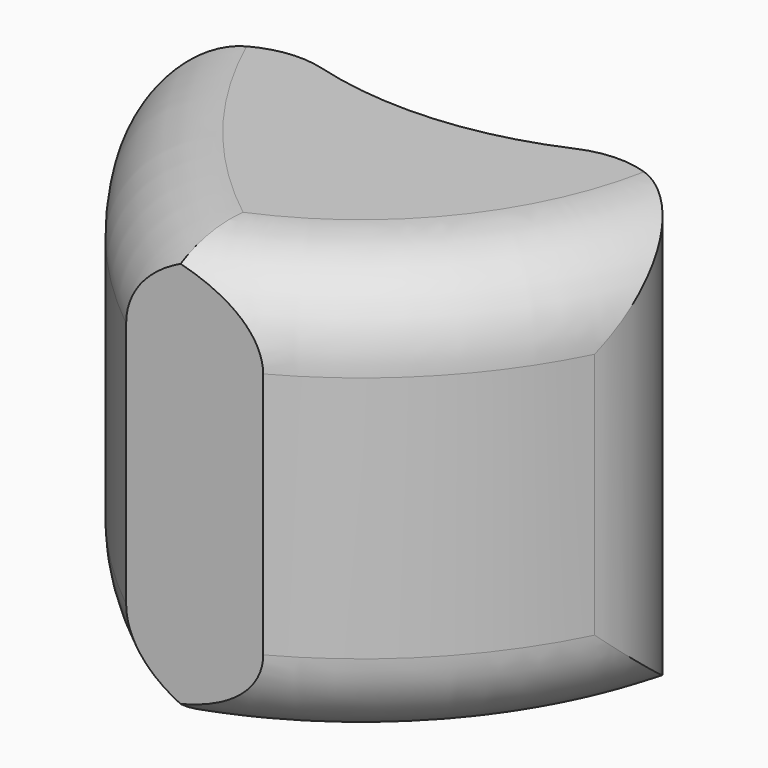
from build123d import *

# Parameters (mm, degrees)
F1_DEPTH     = 23.876
F2_T1_DEPTH  = 110.599658452
F2_T3_DEPTH  = 97.7290207292
F2_T6_ANGLE  = 84.0775345573
F2_T8_ANGLE  = 131.5876567491
F2_T10_ANGLE = 131.5876567491
F2_T12_ANGLE = 84.0775345573


# Not quite as in the source:
# - a fillet or chamfer that OpenCascade refuses, or shapes differently, is made with other operations: its cross-section is extruded or revolved along the edge and cut away or added


with BuildPart() as f1:
    # F0 (on Top) → F1 (new body)
    with BuildSketch(Plane.XY):
        with BuildLine():
            ThreePointArc((-16.8886538595, 0), (-33.6717544124, -9.3917342028), (-50.4548549652, 0))
            ThreePointArc((-50.4548549652, 0), (-46.0831484668, -13.8741388275), (-36.7328226566, -25.0175204128))
            Line((-36.7328226566, -25.0175204128), (-29.1329286993, -25.0175204128))
            ThreePointArc((-29.1329286993, -25.0175204128), (-19.0105144226, -14.4666076853), (-16.8886538595, 0))
        make_face()
    extrude(amount=-F1_DEPTH)

    # F2: fillet of radius 5.08 on 6 edges, made by hand

    # F2_s2 → F2_t1 (cut)
    with BuildSketch(Plane.XY.offset(-67.237829226)):
        with BuildLine():
            ThreePointArc((-38.9861518203, -8.6610502297), (-44.4536744732, -10.5484087098), (-44.6103785769, -16.3303953767))
            ThreePointArc((-44.6103785769, -16.3303953767), (-48.4959513119, -8.5099649673), (-50.4548549652, 0))
            ThreePointArc((-50.4548549652, 0), (-45.5388644987, -5.4141743653), (-38.9861518203, -8.6610502297))
        make_face()
    extrude(amount=F2_T1_DEPTH, mode=Mode.SUBTRACT)

    # F2_s4 → F2_t3 (cut)
    with BuildSketch(Plane.XY.offset(-60.8025103646)):
        with BuildLine():
            ThreePointArc((-19.0798772238, -14.6071656046), (-19.9573949525, -8.8324154802), (-25.6877196822, -7.7005343667))
            ThreePointArc((-25.6877196822, -7.7005343667), (-20.7034351336, -4.5184374558), (-16.8886538595, 0))
            ThreePointArc((-16.8886538595, 0), (-16.8326353552, -7.4763390399), (-19.0798772238, -14.6071656046))
        make_face()
    extrude(amount=F2_T3_DEPTH, mode=Mode.SUBTRACT)

    # F2_s5 → F2_t6 (revolve, cut)
    with BuildSketch(Plane(origin=(0.1965344141, 0.8317793395, 0), x_dir=(0, 0, 1), z_dir=(0.2299501287, 0.9732024138, 0))):
        with BuildLine():
            ThreePointArc((-5.08, -51.2464457493), (-1.4878975516, -49.7585481977), (0, -46.1664457493))
            Line((0, -46.1664457493), (0, -51.2464457493))
            Line((0, -51.2464457493), (-5.08, -51.2464457493))
        make_face()
    revolve(axis=Axis((-13.4102859167, 4.0468248863, 0), (0, 0, 1)), revolution_arc=F2_T6_ANGLE, mode=Mode.SUBTRACT)

    # F2_s7 → F2_t8 (revolve, cut)
    with BuildSketch(Plane(origin=(-40.3967670298, 1.3205110393, 0), x_dir=(0, 0, 1), z_dir=(-0.9994661577, 0.0326710822, 0))):
        with BuildLine():
            ThreePointArc((-5.08, -29.2399824093), (-1.4878975516, -27.7520848577), (0, -24.1599824093))
            Line((0, -24.1599824093), (0, -29.2399824093))
            Line((0, -29.2399824093), (-5.08, -29.2399824093))
        make_face()
    revolve(axis=Axis((-40.5679344471, -3.9158028389, 0), (0, 0, 1)), revolution_arc=F2_T8_ANGLE, mode=Mode.SUBTRACT)

    # F2_s9 → F2_t10 (revolve, cut)
    with BuildSketch(Plane(origin=(-40.3967670298, 1.3205110393, 0), x_dir=(0, 0, 1), z_dir=(-0.9994661577, 0.0326710822, 0))):
        with BuildLine():
            ThreePointArc((-18.796, -29.2399824093), (-22.3881024484, -27.7520848577), (-23.876, -24.1599824093))
            Line((-23.876, -24.1599824093), (-23.876, -29.2399824093))
            Line((-23.876, -29.2399824093), (-18.796, -29.2399824093))
        make_face()
    revolve(axis=Axis((-40.5679344471, -3.9158028389, -23.876), (0, 0, 1)), revolution_arc=F2_T10_ANGLE, mode=Mode.SUBTRACT)

    # F2_s11 → F2_t12 (revolve, cut)
    with BuildSketch(Plane(origin=(0.1965344141, 0.8317793395, 0), x_dir=(0, 0, 1), z_dir=(0.2299501287, 0.9732024138, 0))):
        with BuildLine():
            ThreePointArc((-18.796, -51.2464457493), (-22.3881024484, -49.7585481977), (-23.876, -46.1664457493))
            Line((-23.876, -46.1664457493), (-23.876, -51.2464457493))
            Line((-23.876, -51.2464457493), (-18.796, -51.2464457493))
        make_face()
    revolve(axis=Axis((-13.4102859167, 4.0468248863, -23.876), (0, 0, 1)), revolution_arc=F2_T12_ANGLE, mode=Mode.SUBTRACT)


solid = f1.part
